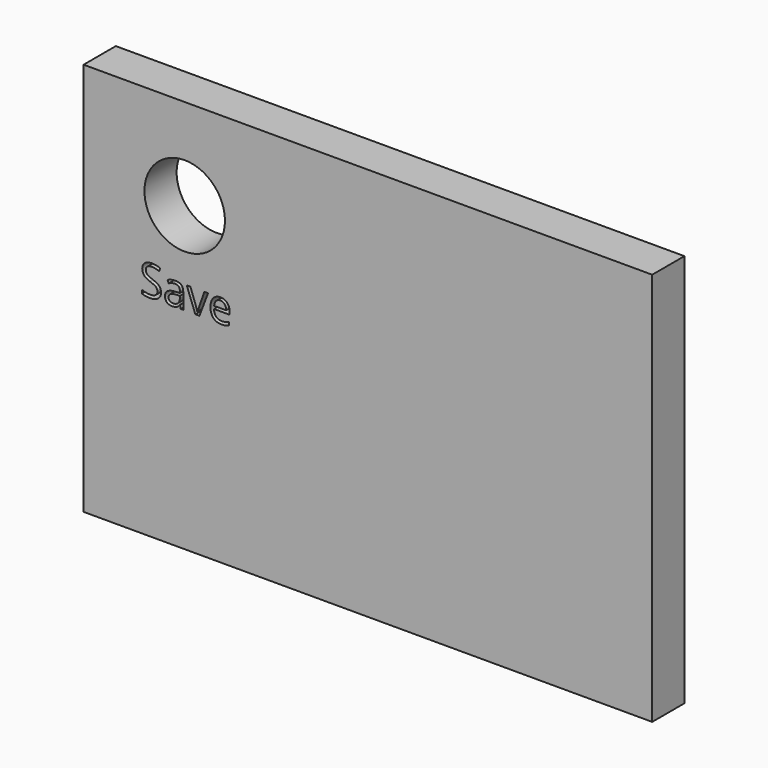
from build123d import *

# Parameters (mm, degrees)
F0_W         = 70.62156127
F0_H         = 48.8975878318
F0_R         = 5
F1_DEPTH     = 5
F2_DEPTH     = 5.001
F3_TEXT_SIZE = 5.2916666667
F4_DEPTH     = 2


# Not quite as in the source:
# - Text() gives the source's letters only with a copy of the font that has no kerning and outlines rounded to 1/6400 em; it was checked with that copy


with BuildPart() as f1:
    # F0 (on Front) → F1 (new body)
    with BuildSketch(Plane.XZ):
        with Locations((35.310780635, 24.4487939159)):
            Rectangle(F0_W, F0_H)
        with Locations((12.5561042132, 37.5419172448)):
            Circle(F0_R, mode=Mode.SUBTRACT)
    extrude(amount=F1_DEPTH)

    # F0 (on Front) → F2 (cut, through all)
    with BuildSketch(Plane.XZ):
        with Locations((12.5561042132, 37.5419172448)):
            Circle(F0_R)
    extrude(amount=F2_DEPTH, mode=Mode.SUBTRACT)

    # F3 (on face) → F4 (cut)
    with BuildSketch(Plane.XZ.offset(5)):
        with Locations((6.9609935361, 26.1119172448)):
            Text('Save', F3_TEXT_SIZE, font='Open Sans', text_align=(TextAlign.LEFT, TextAlign.BOTTOM))
    extrude(amount=-F4_DEPTH, mode=Mode.SUBTRACT)


solid = f1.part
